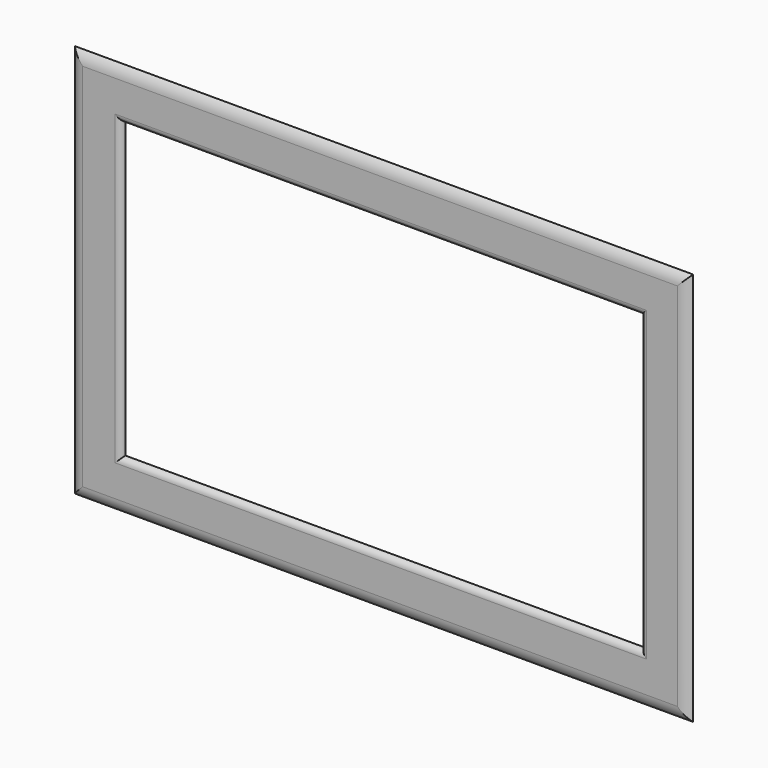
from build123d import *

# Parameters (mm, degrees)
F0_W         = 15.2291797996
F0_H         = 88.5
F0_W_2       = 14.7708202004
F1_DEPTH     = 1.5
F2_T1_DEPTH  = 88.5
F2_T3_DEPTH  = 156
F2_T9_DEPTH  = 93.3412291828
F2_T13_DEPTH = 160.8412291828
F2_T20_DEPTH = 93.3412291828
F2_T24_DEPTH = 160.8412291828
F2_T31_DEPTH = 160.8412291828
F2_T35_DEPTH = 93.3412291828
F2_T42_DEPTH = 93.3412291828
F2_T46_DEPTH = 160.8412291828
F3_T1_DEPTH  = 203.8535710714
F3_T3_DEPTH  = 136.3535710714


# Not quite as in the source:
# - a fillet or chamfer that OpenCascade refuses, or shapes differently, is made with other operations: its cross-section is extruded or revolved along the edge and cut away or added


with BuildPart() as f1:
    # F0 (on Front) → F1 (new body)
    with BuildSketch(Plane.XZ):
        with Locations((-70.9603581131, 10.6903343201)):
            Rectangle(F0_W, F0_H)
        with Locations((100.0396418869, 10.6903343201)):
            Rectangle(F0_W_2, F0_H)
        Polygon((-78.5749480128, 54.9403343201), (-63.3457682133, 54.9403343201), (92.4250519872, 54.9403343201), (92.6542317867, 54.9403343201), (107.4250519872, 54.9403343201), (107.4250519872, 69.9403343201), (107.4249148369, 69.9403343201), (92.6542317867, 69.9403343201), (-63.3457682133, 69.9403343201), (-78.5749480128, 69.9403343201), (-78.5749480128, 64.060893178), align=None)
        Polygon((92.6542317867, -33.5596656799), (-63.3457682133, -33.5596656799), (-78.5749480128, -33.5596656799), (-78.5749480128, -40.4141508043), (-78.5749480128, -48.5596656799), (-63.5749480128, -48.5596656799), (-63.3457682133, -48.5596656799), (92.6542317867, -48.5596656799), (107.4250519872, -48.5596656799), (107.4250519872, -33.5596656799), align=None)
    extrude(amount=F1_DEPTH)

    # F2: fillet of radius 2 on 4 edges, made by hand

    # F2_s2 → F2_t1 (cut)
    with BuildSketch(Plane.XY.offset(-33.5596656799)):
        with BuildLine():
            ThreePointArc((-63.3457682133, 0), (-64.057515015, -1.0811388301), (-65.2822598864, -1.5))
            Line((-65.2822598864, -1.5), (-63.3457682133, -1.5))
            Line((-63.3457682133, -1.5), (-63.3457682133, 0))
        make_face()
        with BuildLine():
            ThreePointArc((92.6542317867, 0), (93.3659785884, -1.0811388301), (94.5907234598, -1.5))
            Line((94.5907234598, -1.5), (92.6542317867, -1.5))
            Line((92.6542317867, -1.5), (92.6542317867, 0))
        make_face()
    extrude(amount=F2_T1_DEPTH, mode=Mode.SUBTRACT)

    # F2_s4 → F2_t3 (cut)
    with BuildSketch(Plane.YZ.offset(-63.3457682133)):
        with BuildLine():
            ThreePointArc((0, 54.9403343201), (-1.0811388301, 55.6520811218), (-1.5, 56.8768259932))
            Line((-1.5, 56.8768259932), (-1.5, 54.9403343201))
            Line((-1.5, 54.9403343201), (0, 54.9403343201))
        make_face()
        with BuildLine():
            ThreePointArc((0, -33.5596656799), (-1.0811388301, -34.2714124816), (-1.5, -35.496157353))
            Line((-1.5, -35.496157353), (-1.5, -33.5596656799))
            Line((-1.5, -33.5596656799), (0, -33.5596656799))
        make_face()
    extrude(amount=F2_T3_DEPTH, mode=Mode.SUBTRACT)


with BuildPart() as f2_tool7:
    # F2_s8 → F2_t9 (new body)
    with BuildSketch(Plane.XY.offset(-38.4008948627)):
        with BuildLine():
            ThreePointArc((-63.3457682133, 0), (-64.057515015, -1.0811388301), (-65.2822598864, -1.5))
            Line((-65.2822598864, -1.5), (-63.3457682133, -1.5))
            Line((-63.3457682133, -1.5), (-63.3457682133, 0))
        make_face()
    extrude(amount=F2_T9_DEPTH)

    split(bisect_by=Plane.XY.offset(-33.5596656799), keep=Keep.BOTTOM)


with BuildPart() as f2_tool11:
    # F2_s12 → F2_t13 (new body)
    with BuildSketch(Plane.YZ.offset(92.6542317867)):
        with BuildLine():
            ThreePointArc((0, -33.5596656799), (-1.0811388301, -34.2714124816), (-1.5, -35.496157353))
            Line((-1.5, -35.496157353), (-1.5, -33.5596656799))
            Line((-1.5, -33.5596656799), (0, -33.5596656799))
        make_face()
    extrude(amount=-F2_T13_DEPTH)

    split(bisect_by=Plane.YZ.offset(-63.3457682133), keep=Keep.BOTTOM)


with BuildPart() as f2_tool7_1:
    add(f2_tool7.part)

    # F2_t15: intersect F2_tool11
    add(f2_tool11.part, mode=Mode.INTERSECT)


with BuildPart() as f1_1:
    add(f1.part)

    # F2_t5: cut F2_tool7
    add(f2_tool7_1.part, mode=Mode.SUBTRACT)


with BuildPart() as f2_tool18:
    # F2_s19 → F2_t20 (new body)
    with BuildSketch(Plane.XY.offset(-33.5596656799)):
        with BuildLine():
            ThreePointArc((-63.3457682133, 0), (-64.057515015, -1.0811388301), (-65.2822598864, -1.5))
            Line((-65.2822598864, -1.5), (-63.3457682133, -1.5))
            Line((-63.3457682133, -1.5), (-63.3457682133, 0))
        make_face()
    extrude(amount=F2_T20_DEPTH)

    split(bisect_by=Plane.XY.offset(54.9403343201), keep=Keep.TOP)


with BuildPart() as f2_tool22:
    # F2_s23 → F2_t24 (new body)
    with BuildSketch(Plane.YZ.offset(-68.186997396)):
        with BuildLine():
            ThreePointArc((0, 54.9403343201), (-1.0811388301, 55.6520811218), (-1.5, 56.8768259932))
            Line((-1.5, 56.8768259932), (-1.5, 54.9403343201))
            Line((-1.5, 54.9403343201), (0, 54.9403343201))
        make_face()
    extrude(amount=F2_T24_DEPTH)

    split(bisect_by=Plane.YZ.offset(-63.3457682133), keep=Keep.BOTTOM)


with BuildPart() as f2_tool18_1:
    add(f2_tool18.part)

    # F2_t26: intersect F2_tool22
    add(f2_tool22.part, mode=Mode.INTERSECT)


with BuildPart() as f1_2:
    add(f1_1.part)

    # F2_t16: cut F2_tool18
    add(f2_tool18_1.part, mode=Mode.SUBTRACT)


with BuildPart() as f2_tool29:
    # F2_s30 → F2_t31 (new body)
    with BuildSketch(Plane.YZ.offset(-63.3457682133)):
        with BuildLine():
            ThreePointArc((0, 54.9403343201), (-1.0811388301, 55.6520811218), (-1.5, 56.8768259932))
            Line((-1.5, 56.8768259932), (-1.5, 54.9403343201))
            Line((-1.5, 54.9403343201), (0, 54.9403343201))
        make_face()
    extrude(amount=F2_T31_DEPTH)

    split(bisect_by=Plane.YZ.offset(92.6542317867), keep=Keep.TOP)


with BuildPart() as f2_tool33:
    # F2_s34 → F2_t35 (new body)
    with BuildSketch(Plane.XY.offset(59.7815635028)):
        with BuildLine():
            ThreePointArc((92.6542317867, 0), (93.3659785884, -1.0811388301), (94.5907234598, -1.5))
            Line((94.5907234598, -1.5), (92.6542317867, -1.5))
            Line((92.6542317867, -1.5), (92.6542317867, 0))
        make_face()
    extrude(amount=-F2_T35_DEPTH)

    split(bisect_by=Plane.XY.offset(54.9403343201), keep=Keep.TOP)


with BuildPart() as f2_tool29_1:
    add(f2_tool29.part)

    # F2_t37: intersect F2_tool33
    add(f2_tool33.part, mode=Mode.INTERSECT)


with BuildPart() as f1_3:
    add(f1_2.part)

    # F2_t27: cut F2_tool29
    add(f2_tool29_1.part, mode=Mode.SUBTRACT)


with BuildPart() as f2_tool40:
    # F2_s41 → F2_t42 (new body)
    with BuildSketch(Plane.XY.offset(54.9403343201)):
        with BuildLine():
            ThreePointArc((92.6542317867, 0), (93.3659785884, -1.0811388301), (94.5907234598, -1.5))
            Line((94.5907234598, -1.5), (92.6542317867, -1.5))
            Line((92.6542317867, -1.5), (92.6542317867, 0))
        make_face()
    extrude(amount=-F2_T42_DEPTH)

    split(bisect_by=Plane.XY.offset(-33.5596656799), keep=Keep.BOTTOM)


with BuildPart() as f2_tool44:
    # F2_s45 → F2_t46 (new body)
    with BuildSketch(Plane.YZ.offset(97.4954609695)):
        with BuildLine():
            ThreePointArc((0, -33.5596656799), (-1.0811388301, -34.2714124816), (-1.5, -35.496157353))
            Line((-1.5, -35.496157353), (-1.5, -33.5596656799))
            Line((-1.5, -33.5596656799), (0, -33.5596656799))
        make_face()
    extrude(amount=-F2_T46_DEPTH)

    split(bisect_by=Plane.YZ.offset(92.6542317867), keep=Keep.TOP)


with BuildPart() as f2_tool40_1:
    add(f2_tool40.part)

    # F2_t48: intersect F2_tool44
    add(f2_tool44.part, mode=Mode.INTERSECT)


with BuildPart() as f1_4:
    add(f1_3.part)

    # F2_t38: cut F2_tool40
    add(f2_tool40_1.part, mode=Mode.SUBTRACT)

    # F3: fillet of radius 5 on 4 edges, made by hand

    # F3_s2 → F3_t1 (cut)
    with BuildSketch(Plane.YZ.offset(-87.5017335485)):
        with BuildLine():
            ThreePointArc((-1.5, 66.3696201058), (-1.1097722286, 68.3061117789), (0, 69.9403343201))
            Line((0, 69.9403343201), (-1.5, 69.9403343201))
            Line((-1.5, 69.9403343201), (-1.5, 66.3696201058))
        make_face()
        with BuildLine():
            ThreePointArc((-1.5, -44.9889514657), (-1.1097722286, -46.9254431388), (0, -48.5596656799))
            Line((0, -48.5596656799), (-1.5, -48.5596656799))
            Line((-1.5, -48.5596656799), (-1.5, -44.9889514657))
        make_face()
    extrude(amount=F3_T1_DEPTH, mode=Mode.SUBTRACT)

    # F3_s4 → F3_t3 (cut)
    with BuildSketch(Plane.XY.offset(-57.4864512156)):
        with BuildLine():
            ThreePointArc((103.8543377729, -1.5), (105.790829446, -1.1097722286), (107.4250519872, 0))
            Line((107.4250519872, 0), (107.4250519872, -1.5))
            Line((107.4250519872, -1.5), (103.8543377729, -1.5))
        make_face()
        with BuildLine():
            ThreePointArc((-75.0042337986, -1.5), (-76.9407254717, -1.1097722286), (-78.5749480128, 0))
            Line((-78.5749480128, 0), (-78.5749480128, -1.5))
            Line((-78.5749480128, -1.5), (-75.0042337986, -1.5))
        make_face()
    extrude(amount=F3_T3_DEPTH, mode=Mode.SUBTRACT)


solid = f1_4.part
